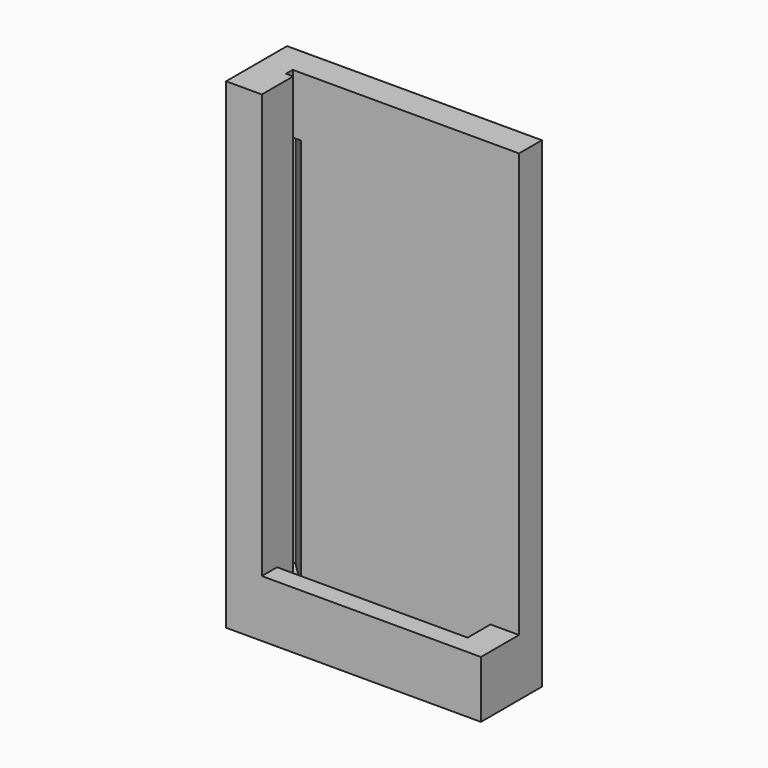
from build123d import *

# Parameters (mm, degrees)
F1_DEPTH = 25
F2_DEPTH = 165
F4_DEPTH = 190
F5_W     = 12
F5_H     = 8
F5_H_2   = 12
F6_DEPTH = 12
F7_W     = 107
F7_H     = 32
F8_DEPTH = 12


with BuildPart() as f1:
    # F0 (on Top) → F1 (new body)
    with BuildSketch(Plane.XY):
        Polygon((-15.4107665035, -11.7272357842), (-11.8752325976, -15.2627696901), (79.5892334965, -15.2627696901), (79.5892334965, -3.2627696901), (-15.4107665035, -3.2627696901), align=None)
        Polygon((-23.8752325976, -3.2627696901), (-15.4107665035, -11.7272357842), (-15.4107665035, -3.2627696901), align=None)
        Polygon((-18.9463004094, -15.2627696901), (-15.4107665035, -15.2627696901), (-27.4107665035, -3.2627696901), (-27.4107665035, -6.7983035961), align=None)
        Polygon((-27.4107665035, -15.2627696901), (-18.9463004094, -15.2627696901), (-27.4107665035, -6.7983035961), align=None)
        Polygon((-15.4107665035, -18.7983035961), (-18.9463004094, -15.2627696901), (-27.4107665035, -15.2627696901), (-27.4107665035, -35.2627696901), (-15.4107665035, -35.2627696901), align=None)
        Polygon((-27.4107665035, -3.2627696901), (-15.4107665035, -15.2627696901), (-15.4107665035, -11.7272357842), (-23.8752325976, -3.2627696901), align=None)
        Polygon((-15.4107665035, -11.7272357842), (-15.4107665035, -15.2627696901), (-11.8752325976, -15.2627696901), align=None)
        Polygon((-15.4107665035, -18.7983035961), (-15.4107665035, -15.2627696901), (-18.9463004094, -15.2627696901), align=None)
    extrude(amount=F1_DEPTH)

    # F0 (on Top) → F2 (join)
    with BuildSketch(Plane.XY):
        Polygon((-15.4107665035, -18.7983035961), (-18.9463004094, -15.2627696901), (-27.4107665035, -15.2627696901), (-27.4107665035, -35.2627696901), (-15.4107665035, -35.2627696901), align=None)
        Polygon((-23.8752325976, -3.2627696901), (-15.4107665035, -11.7272357842), (-15.4107665035, -3.2627696901), align=None)
        Polygon((-15.4107665035, -11.7272357842), (-11.8752325976, -15.2627696901), (79.5892334965, -15.2627696901), (79.5892334965, -3.2627696901), (-15.4107665035, -3.2627696901), align=None)
        Polygon((-27.4107665035, -15.2627696901), (-18.9463004094, -15.2627696901), (-27.4107665035, -6.7983035961), align=None)
    extrude(amount=-F2_DEPTH)

    # F3 (on face) → F4 (join, through all)
    with BuildSketch(Plane(origin=(0, 0, -165), x_dir=(1, 0, 0), z_dir=(0, 0, -1))):
        Polygon((-15.4107665035, 30.7983035961), (-15.4107665035, 18.7983035961), (-12.4107665035, 18.7983035961), (-12.4107665035, 30.7983035961), (-12.4107665035, 35.2627696901), (-15.4107665035, 35.2627696901), align=None)
    extrude(amount=-F4_DEPTH)

    # F5 (on face) → F6 (join)
    with BuildSketch(Plane(origin=(0, 0, -165), x_dir=(1, 0, 0), z_dir=(0, 0, -1))):
        Polygon((-12.4107665035, 35.2627696901), (-12.4107665035, 30.7983035961), (-12.4107665035, 27.2627696901), (67.5892334965, 27.2627696901), (67.5892334965, 35.2627696901), align=None)
        with Locations((73.5892334965, 31.2627696901)):
            Rectangle(F5_W, F5_H)
        with Locations((73.5892334965, 21.2627696901)):
            Rectangle(F5_W, F5_H_2)
        Polygon((79.5892334965, 15.2627696901), (67.5892334965, 15.2627696901), (-11.8752325976, 15.2627696901), (-23.8752325976, 3.2627696901), (79.5892334965, 3.2627696901), align=None)
    extrude(amount=-F6_DEPTH)

    # F7 (on face) → F8 (join)
    with BuildSketch(Plane(origin=(0, 0, -165), x_dir=(1, 0, 0), z_dir=(0, 0, -1))):
        with Locations((26.0892334965, 19.2627696901)):
            Rectangle(F7_W, F7_H)
    extrude(amount=F8_DEPTH)


solid = f1.part
